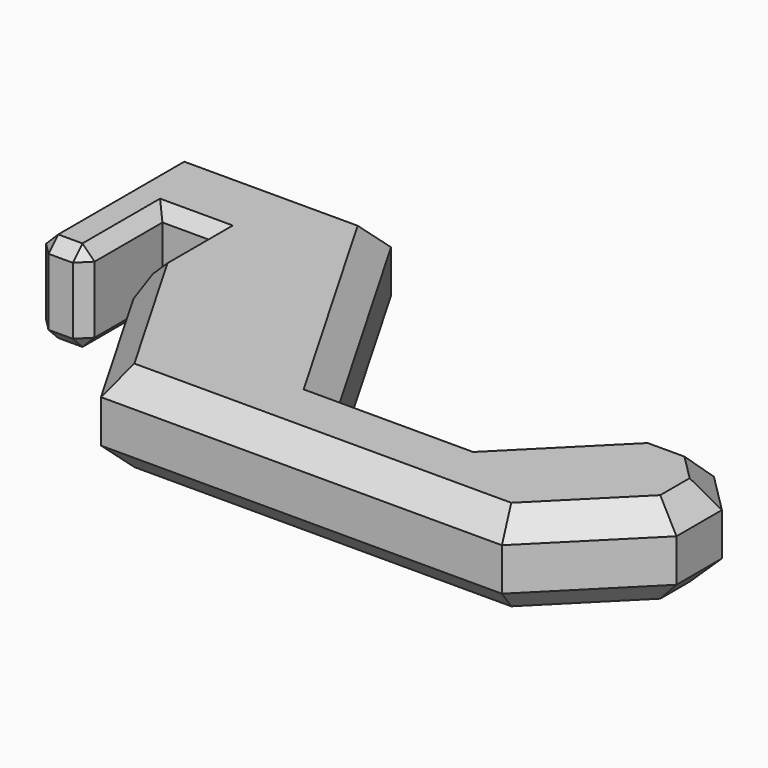
from build123d import *

# Parameters (mm, degrees)
F1_DEPTH = 5.969
F2_W     = 3.175
F2_H     = 6.35
F3_DEPTH = 5.97
F4_SIZE  = 0.79375
F5_SIZE  = 1.58749


# Not quite as in the source:
# - a fillet or chamfer is up to 0.001 mm smaller than in the source, because OpenCascade refuses the exact size


with BuildPart() as f1:
    # F0 (on Top) → F1 (new body)
    with BuildSketch(Plane.XY):
        Polygon((13.0595644766, 0), (0, 0), (0, -12.7), (6.35, -12.7), (11.849261314, -22.225), (38.1, -22.225), (44.45, -15.875), (44.45, -12.1552561211), (41.8197438789, -9.525), (38.1, -9.525), (31.75, -15.875), (22.225, -15.875), align=None)
    extrude(amount=F1_DEPTH)

    # F2 (on face) → F3 (cut, through all)
    with BuildSketch(Plane.XY.offset(5.969)):
        with Locations((4.7625, -9.525)):
            Rectangle(F2_W, F2_H)
    extrude(amount=-F3_DEPTH, mode=Mode.SUBTRACT)

    # F4
    f4_edges = [f1.edges().sort_by_distance(p)[0] for p in [
        (0, 0, 2.9845),
        (0, -12.7, 2.9845),
        (0, -6.35, 0),
        (0, -6.35, 5.969),
        (1.5875, -12.7, 0),
        (3.175, -12.7, 2.9845),
        (1.5875, -12.7, 5.969),
        (3.175, -9.525, 5.969),
        (3.175, -9.525, 0),
        (4.7625, -6.35, 5.969),
        (6.35, -9.525, 5.969),
        (4.7625, -6.35, 0),
        (6.35, -9.525, 0),
    ]]
    chamfer(f4_edges, length=F4_SIZE)

    # F5 (size 1.5875 in the source; OpenCascade refuses exactly that, so slightly less here)
    f5_edges = [f1.edges().sort_by_distance(p)[0] for p in [
        (6.926657, 0, 0),
        (17.642282, -7.9375, 0),
        (26.9875, -15.875, 0),
        (34.925, -12.7, 0),
        (39.959872, -9.525, 0),
        (43.134872, -10.840128, 0),
        (44.45, -14.015128, 0),
        (41.275, -19.05, 0),
        (24.974631, -22.225, 0),
        (9.496506, -18.149908, 0),
        (9.496506, -18.149908, 5.969),
        (24.974631, -22.225, 5.969),
        (41.275, -19.05, 5.969),
        (44.45, -14.015128, 5.969),
        (43.134872, -10.840128, 5.969),
        (34.925, -12.7, 5.969),
        (39.959872, -9.525, 5.969),
        (26.9875, -15.875, 5.969),
        (17.642282, -7.9375, 5.969),
        (6.926657, 0, 5.969),
    ]]
    chamfer(f5_edges, length=F5_SIZE)


solid = f1.part
